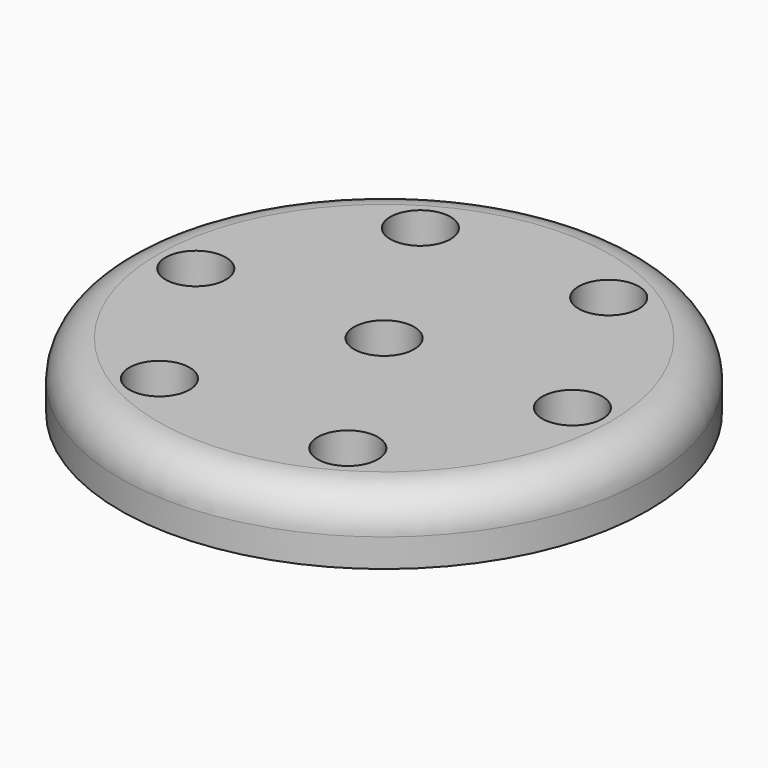
from build123d import *

# Parameters (mm, degrees)
F0_R     = 14.0159979079
F0_R_2   = 1.6
F1_DEPTH = 3.5
F2_R     = 2


# Not quite as in the source:
# - a feature names something its author has since deleted; it is built from what else it names


with BuildPart() as f1:
    # F0 (on Top) → F1 (new body)
    with BuildSketch(Plane.XY):
        with Locations((4.1739126741, 0)):
            Circle(F0_R)
        with Locations((-0.8260871004, -8.6602539076)):
            Circle(F0_R_2, mode=Mode.SUBTRACT)
        with Locations((-5.8260870252, 0)):
            Circle(F0_R_2, mode=Mode.SUBTRACT)
        with Locations((4.1739126741, 0)):
            Circle(F0_R_2, mode=Mode.SUBTRACT)
        with Locations((9.1739127493, -8.6602539076)):
            Circle(F0_R_2, mode=Mode.SUBTRACT)
        with Locations((14.1739126741, 0)):
            Circle(F0_R_2, mode=Mode.SUBTRACT)
        with Locations((-0.8260871004, 8.6602539076)):
            Circle(F0_R_2, mode=Mode.SUBTRACT)
        with Locations((9.1739127493, 8.6602539076)):
            Circle(F0_R_2, mode=Mode.SUBTRACT)
    extrude(amount=F1_DEPTH)

    # F2
    f2_edges = [f1.edges().sort_by_distance(p)[0] for p in [
        (-9.842085, 0, 3.5),
    ]]
    fillet(f2_edges, radius=F2_R)


solid = f1.part
